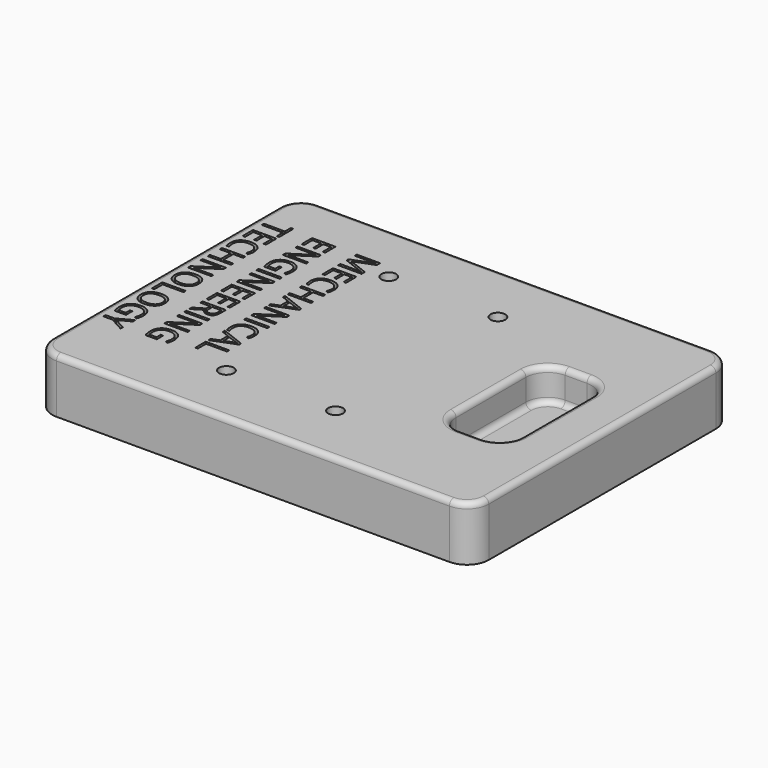
from build123d import *

# Parameters (mm, degrees)
F1_DEPTH       = 50
F2_DEPTH       = 20
F3_D           = 13.5
F3_CBORE_D     = 23.78
F3_CBORE_DEPTH = 7.95
F4_TEXT_SIZE   = 30.0236905683
F5_DEPTH       = 5
F6_R           = 5


# Not quite as in the source:
# - Text() gives the source's letters only with a copy of the font that has no kerning and outlines rounded to 1/6400 em; it was checked with that copy


with BuildPart() as f1:
    # F0 (on Top) → F1 (new body)
    with BuildSketch(Plane.XY):
        with BuildLine():
            Line((-180, -150), (180, -150))
            ThreePointArc((180, -150), (194.1421356237, -144.1421356237), (200, -130))
            Line((200, -130), (200, 130))
            ThreePointArc((200, 130), (194.1421356237, 144.1421356237), (180, 150))
            Line((180, 150), (-180, 150))
            ThreePointArc((-180, 150), (-194.1421356237, 144.1421356237), (-200, 130))
            Line((-200, 130), (-200, -130))
            ThreePointArc((-200, -130), (-194.1421356237, -144.1421356237), (-180, -150))
        make_face()
        with BuildLine():
            ThreePointArc((158, -40), (152.1421356237, -54.1421356237), (138, -60))
            Line((138, -60), (118, -60))
            ThreePointArc((118, -60), (103.8578643763, -54.1421356237), (98, -40))
            Line((98, -40), (98, 40))
            ThreePointArc((98, 40), (103.8578643763, 54.1421356237), (118, 60))
            Line((118, 60), (138, 60))
            ThreePointArc((138, 60), (152.1421356237, 54.1421356237), (158, 40))
            Line((158, 40), (158, -40))
        make_face(mode=Mode.SUBTRACT)
    extrude(amount=F1_DEPTH)

    # F0 (on Top) → F2 (join)
    with BuildSketch(Plane.XY):
        with BuildLine():
            Line((118, -60), (138, -60))
            ThreePointArc((138, -60), (152.1421356237, -54.1421356237), (158, -40))
            Line((158, -40), (158, 40))
            ThreePointArc((158, 40), (152.1421356237, 54.1421356237), (138, 60))
            Line((138, 60), (118, 60))
            ThreePointArc((118, 60), (103.8578643763, 54.1421356237), (98, 40))
            Line((98, 40), (98, -40))
            ThreePointArc((98, -40), (103.8578643763, -54.1421356237), (118, -60))
        make_face()
    extrude(amount=F2_DEPTH)

    # F3 (through all)
    with Locations(Plane(origin=(0, 0, 0), x_dir=(1, 0, 0), z_dir=(0, 0, -1))):
        with Locations((-70, 93), (30, 93), (30, -93), (-70, -93)):
            CounterBoreHole(F3_D / 2, F3_CBORE_D / 2, F3_CBORE_DEPTH)

    # F4 (on face) → F5 (cut)
    with BuildSketch(Plane.XY.offset(50)):
        with Locations(Location((-109.3828827143, 108.3829402924), (0, 0, -90))):
            Text('MECHANICAL', F4_TEXT_SIZE, font='Open Sans', text_align=(TextAlign.LEFT, TextAlign.BOTTOM))
        with Locations(Location((-150.2151018872, 108.3829402924), (0, 0, -90))):
            Text('ENGINEERING', F4_TEXT_SIZE, font='Open Sans', text_align=(TextAlign.LEFT, TextAlign.BOTTOM))
        with Locations(Location((-191.0473210602, 108.3829402924), (0, 0, -90))):
            Text('TECHNOLOGY', F4_TEXT_SIZE, font='Open Sans', text_align=(TextAlign.LEFT, TextAlign.BOTTOM))
    extrude(amount=-F5_DEPTH, mode=Mode.SUBTRACT)

    # F6
    f6_edges = [f1.edges().sort_by_distance(p)[0] for p in [
        (0, -150, 50),
        (158, 0, 50),
        (158, 0, 20),
    ]]
    fillet(f6_edges, radius=F6_R)


solid = f1.part
